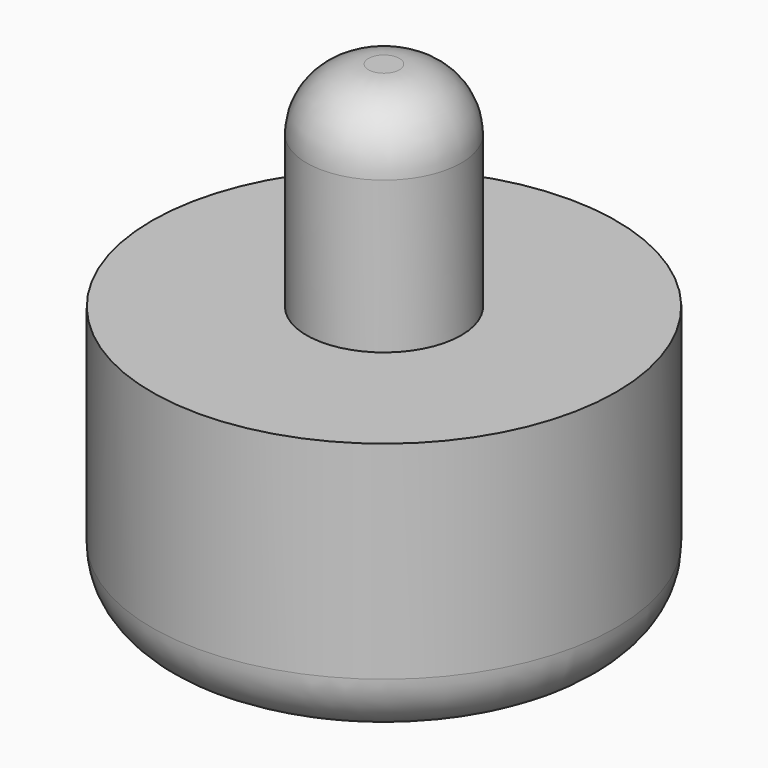
from build123d import *

# Parameters (mm, degrees)
F0_R     = 9.525
F1_DEPTH = 11.049
F2_R     = 2.54
F3_R     = 3.175
F4_DEPTH = 8.763
F5_R     = 2.54


# Not quite as in the source:
# - a feature names something its author has since deleted; it is built from what else it names


with BuildPart() as f1:
    # F0 (on Top) → F1 (new body)
    with BuildSketch(Plane.XY):
        with Locations((-0.0108847216, 0.0162923955)):
            Circle(F0_R)
    extrude(amount=F1_DEPTH)

    # F2
    f2_edges = [f1.edges().sort_by_distance(p)[0] for p in [
        (-9.535885, 0.016292, 0),
    ]]
    fillet(f2_edges, radius=F2_R)

    # F3 (on face) → F4 (join)
    with BuildSketch(Plane.XY.offset(11.049)):
        Circle(F3_R)
    extrude(amount=F4_DEPTH)

    # F5
    f5_edges = [f1.edges().sort_by_distance(p)[0] for p in [
        (-3.175, 0, 19.812),
    ]]
    fillet(f5_edges, radius=F5_R)


solid = f1.part
